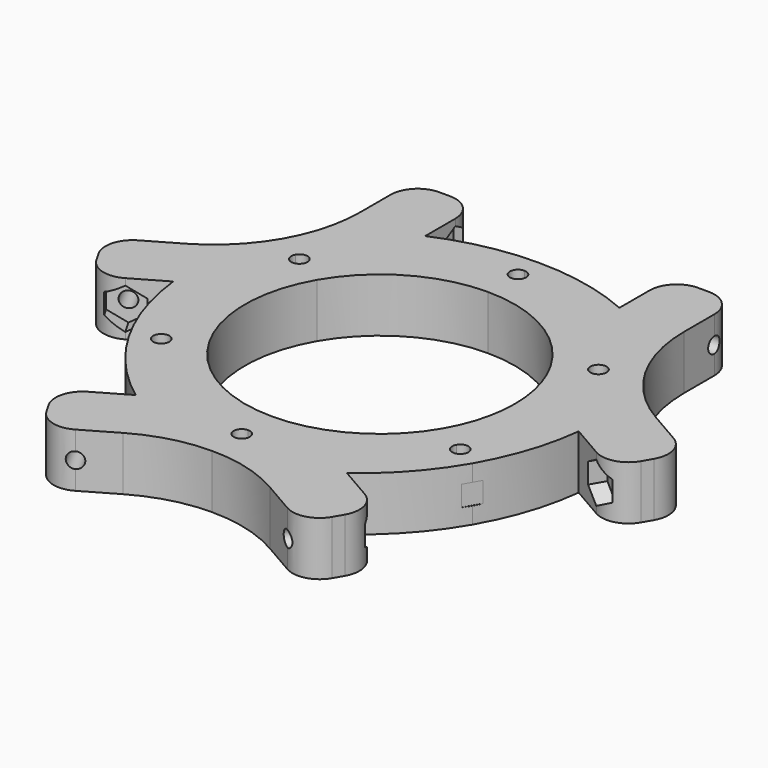
from build123d import *

# Parameters (mm, degrees)
F1_DEPTH      = 10
F2_R          = 1.45
F3_DEPTH      = 30
F3_DEPTH_BACK = 30
F4_ANGLE      = 120
F5_ANGLE      = 120
F7_T1_DEPTH   = 35
F8_DEPTH      = 21
F8_DEPTH_BACK = 21
F9_ANGLE      = 120
F10_ANGLE     = 120


# Not quite as in the source:
# - a fillet or chamfer that OpenCascade refuses, or shapes differently, is made with other operations: its cross-section is extruded or revolved along the edge and cut away or added
# - a feature names something its author has since deleted; it is built from what else it names


with BuildPart() as f1:
    # F0 (on Top) → F1 (new body)
    with BuildSketch(Plane.XY):
        with BuildLine():
            ThreePointArc((-21.6506350946, 12.5), (-12.5, 21.6506350946), (0, 25))
            Line((0, 25), (0, 30.5))
            ThreePointArc((0, 30.5), (-1.5, 32), (0, 33.5))
            Line((0, 33.5), (0, 36.7568187454))
            ThreePointArc((0, 36.7568187454), (-9.193933966, 35.8076028273), (-18, 33))
            Line((-18, 33), (-18, 45))
            Line((-18, 45), (-30, 45))
            Line((-30, 45), (-30, 33))
            ThreePointArc((-30, 33), (-30.9253753917, 25.9710760623), (-33.6384387633, 19.4211616751))
            Line((-33.6384387633, 19.4211616751), (-29.0118510268, 16.75))
            ThreePointArc((-29.0118510268, 16.75), (-27.3245843534, 17.4488887394), (-26.2128129211, 16))
            ThreePointArc((-26.2128129211, 16), (-26.2639241817, 15.6117714323), (-26.4137748154, 15.25))
            Line((-26.4137748154, 15.25), (-21.6506350946, 12.5))
        make_face()
        with BuildLine():
            ThreePointArc((0, -25), (-12.5, -21.6506350946), (-21.6506350946, -12.5))
            Line((-21.6506350946, -12.5), (-26.4137748154, -15.25))
            ThreePointArc((-26.4137748154, -15.25), (-26.2639241817, -15.6117714323), (-26.2128129211, -16))
            ThreePointArc((-26.2128129211, -16), (-27.3245843534, -17.4488887394), (-29.0118510268, -16.75))
            Line((-29.0118510268, -16.75), (-31.8323387958, -18.3784093727))
            ThreePointArc((-31.8323387958, -18.3784093727), (-26.413326714, -25.8659817889), (-19.5788383249, -32.0884572681))
            Line((-19.5788383249, -32.0884572681), (-29.9711431703, -38.0884572681))
            Line((-29.9711431703, -38.0884572681), (-23.9711431703, -48.4807621135))
            Line((-23.9711431703, -48.4807621135), (-13.5788383249, -42.4807621135))
            ThreePointArc((-13.5788383249, -42.4807621135), (-7.0289239377, -39.767698742), (0, -38.8423233502))
            Line((0, -38.8423233502), (0, -33.5))
            ThreePointArc((0, -33.5), (-1.5, -32), (0, -30.5))
            Line((0, -30.5), (0, -25))
        make_face()
        with BuildLine():
            Line((0, 30.5), (0, 25))
            ThreePointArc((0, 25), (12.5, 21.6506350946), (21.6506350946, 12.5))
            Line((21.6506350946, 12.5), (26.4137748154, 15.25))
            ThreePointArc((26.4137748154, 15.25), (26.9628129211, 17.2990381057), (29.0118510268, 16.75))
            Line((29.0118510268, 16.75), (33.6384387633, 19.4211616751))
            ThreePointArc((33.6384387633, 19.4211616751), (30.9253753917, 25.9710760623), (30, 33))
            Line((30, 33), (30, 45))
            Line((30, 45), (18, 45))
            Line((18, 45), (18, 33))
            ThreePointArc((18, 33), (9.193933966, 35.8076028273), (0, 36.7568187454))
            Line((0, 36.7568187454), (0, 33.5))
            ThreePointArc((0, 33.5), (1.0606601718, 33.0606601718), (1.5, 32))
            ThreePointArc((1.5, 32), (1.0606601718, 30.9393398282), (0, 30.5))
        make_face()
        with BuildLine():
            ThreePointArc((25, 0), (24.1481456572, -6.4704761276), (21.6506350946, -12.5))
            Line((21.6506350946, -12.5), (26.4137748154, -15.25))
            ThreePointArc((26.4137748154, -15.25), (28.1010414888, -14.5511112606), (29.2128129211, -16))
            ThreePointArc((29.2128129211, -16), (29.1617016605, -16.3882285677), (29.0118510268, -16.75))
            Line((29.0118510268, -16.75), (31.8323387958, -18.3784093727))
            ThreePointArc((31.8323387958, -18.3784093727), (35.6072606801, -9.9416210384), (37.5788383249, -0.9115427319))
            Line((37.5788383249, -0.9115427319), (47.9711431703, -6.9115427319))
            Line((47.9711431703, -6.9115427319), (53.9711431703, 3.4807621135))
            Line((53.9711431703, 3.4807621135), (43.5788383249, 9.4807621135))
            ThreePointArc((43.5788383249, 9.4807621135), (37.9542993294, 13.7966226797), (33.6384387633, 19.4211616751))
            Line((33.6384387633, 19.4211616751), (29.0118510268, 16.75))
            ThreePointArc((29.0118510268, 16.75), (29.1617016605, 16.3882285677), (29.2128129211, 16))
            ThreePointArc((29.2128129211, 16), (28.1010414888, 14.5511112606), (26.4137748154, 15.25))
            Line((26.4137748154, 15.25), (21.6506350946, 12.5))
            ThreePointArc((21.6506350946, 12.5), (24.1481456572, 6.4704761276), (25, 0))
        make_face()
        with BuildLine():
            Line((-26.4137748154, -15.25), (-21.6506350946, -12.5))
            ThreePointArc((-21.6506350946, -12.5), (-25, 0), (-21.6506350946, 12.5))
            Line((-21.6506350946, 12.5), (-26.4137748154, 15.25))
            ThreePointArc((-26.4137748154, 15.25), (-28.4628129211, 14.7009618943), (-29.0118510268, 16.75))
            Line((-29.0118510268, 16.75), (-33.6384387633, 19.4211616751))
            ThreePointArc((-33.6384387633, 19.4211616751), (-37.9542993294, 13.7966226797), (-43.5788383249, 9.4807621135))
            Line((-43.5788383249, 9.4807621135), (-53.9711431703, 3.4807621135))
            Line((-53.9711431703, 3.4807621135), (-47.9711431703, -6.9115427319))
            Line((-47.9711431703, -6.9115427319), (-37.5788383249, -0.9115427319))
            ThreePointArc((-37.5788383249, -0.9115427319), (-35.6072606801, -9.9416210384), (-31.8323387958, -18.3784093727))
            Line((-31.8323387958, -18.3784093727), (-29.0118510268, -16.75))
            ThreePointArc((-29.0118510268, -16.75), (-28.4628129211, -14.7009618943), (-26.4137748154, -15.25))
        make_face()
        with BuildLine():
            Line((26.4137748154, -15.25), (21.6506350946, -12.5))
            ThreePointArc((21.6506350946, -12.5), (12.5, -21.6506350946), (0, -25))
            Line((0, -25), (0, -30.5))
            ThreePointArc((0, -30.5), (1.0606601718, -30.9393398282), (1.5, -32))
            ThreePointArc((1.5, -32), (1.0606601718, -33.0606601718), (0, -33.5))
            Line((0, -33.5), (0, -38.8423233502))
            ThreePointArc((0, -38.8423233502), (7.0289239377, -39.767698742), (13.5788383249, -42.4807621135))
            Line((13.5788383249, -42.4807621135), (23.9711431703, -48.4807621135))
            Line((23.9711431703, -48.4807621135), (29.9711431703, -38.0884572681))
            Line((29.9711431703, -38.0884572681), (19.5788383249, -32.0884572681))
            ThreePointArc((19.5788383249, -32.0884572681), (26.413326714, -25.8659817889), (31.8323387958, -18.3784093727))
            Line((31.8323387958, -18.3784093727), (29.0118510268, -16.75))
            ThreePointArc((29.0118510268, -16.75), (26.9628129211, -17.2990381057), (26.4137748154, -15.25))
        make_face()
    extrude(amount=F1_DEPTH)


with BuildPart() as f3:
    # F2 (on Right) → F3 (new body, two sides)
    with BuildSketch(Plane.YZ) as f3_sk:
        with Locations((40, 5)):
            Circle(F2_R)
    extrude(amount=F3_DEPTH)
    extrude(f3_sk.sketch, amount=-F3_DEPTH_BACK)


with BuildPart() as f4_1:
    # F4: copy of F3
    add(f3.part.rotate(Axis((0, 0, 10), (0, 0, -1)), F4_ANGLE))


with BuildPart() as f5_1:
    # F5: copy of F4_1
    add(f4_1.part.rotate(Axis((0, 0, 10), (0, 0, -1)), F5_ANGLE))


with BuildPart() as f1_1:
    add(f1.part)

    # F6: cut F5_1, F3, F4_1
    add(f5_1.part, mode=Mode.SUBTRACT)
    add(f3.part, mode=Mode.SUBTRACT)
    add(f4_1.part, mode=Mode.SUBTRACT)

    # F7: fillet of radius 5 on 12 edges, made by hand

    # F7_s2 → F7_t1 (cut)
    with BuildSketch(Plane.XY.offset(-12.5)):
        with BuildLine():
            ThreePointArc((-26.4711431703, -44.1506350946), (-23.4351113769, -46.4802642261), (-19.6410161514, -45.9807621135))
            Line((-19.6410161514, -45.9807621135), (-23.9711431703, -48.4807621135))
            Line((-23.9711431703, -48.4807621135), (-26.4711431703, -44.1506350946))
        make_face()
        with BuildLine():
            ThreePointArc((19.6410161514, -45.9807621135), (23.4351113769, -46.4802642261), (26.4711431703, -44.1506350946))
            Line((26.4711431703, -44.1506350946), (23.9711431703, -48.4807621135))
            Line((23.9711431703, -48.4807621135), (19.6410161514, -45.9807621135))
        make_face()
        with BuildLine():
            ThreePointArc((51.4711431703, -0.8493649054), (51.9706452828, 2.9447303201), (49.6410161514, 5.9807621135))
            Line((49.6410161514, 5.9807621135), (53.9711431703, 3.4807621135))
            Line((53.9711431703, 3.4807621135), (51.4711431703, -0.8493649054))
        make_face()
        with BuildLine():
            ThreePointArc((30, 40), (28.5355339059, 43.5355339059), (25, 45))
            Line((25, 45), (30, 45))
            Line((30, 45), (30, 40))
        make_face()
        with BuildLine():
            ThreePointArc((-25, 45), (-28.5355339059, 43.5355339059), (-30, 40))
            Line((-30, 40), (-30, 45))
            Line((-30, 45), (-25, 45))
        make_face()
        with BuildLine():
            ThreePointArc((-49.6410161514, 5.9807621135), (-51.9706452828, 2.9447303201), (-51.4711431703, -0.8493649054))
            Line((-51.4711431703, -0.8493649054), (-53.9711431703, 3.4807621135))
            Line((-53.9711431703, 3.4807621135), (-49.6410161514, 5.9807621135))
        make_face()
        with BuildLine():
            ThreePointArc((27.4711431703, -42.418584287), (27.9706452828, -38.6244890615), (25.6410161514, -35.5884572681))
            Line((25.6410161514, -35.5884572681), (29.9711431703, -38.0884572681))
            Line((29.9711431703, -38.0884572681), (27.4711431703, -42.418584287))
        make_face()
        with BuildLine():
            ThreePointArc((43.6410161514, -4.4115427319), (47.4351113769, -4.9110448444), (50.4711431703, -2.581415713))
            Line((50.4711431703, -2.581415713), (47.9711431703, -6.9115427319))
            Line((47.9711431703, -6.9115427319), (43.6410161514, -4.4115427319))
        make_face()
        with BuildLine():
            ThreePointArc((23, 45), (19.4644660941, 43.5355339059), (18, 40))
            Line((18, 40), (18, 45))
            Line((18, 45), (23, 45))
        make_face()
        with BuildLine():
            ThreePointArc((-18, 40), (-19.4644660941, 43.5355339059), (-23, 45))
            Line((-23, 45), (-18, 45))
            Line((-18, 45), (-18, 40))
        make_face()
        with BuildLine():
            ThreePointArc((-50.4711431703, -2.581415713), (-47.4351113769, -4.9110448444), (-43.6410161514, -4.4115427319))
            Line((-43.6410161514, -4.4115427319), (-47.9711431703, -6.9115427319))
            Line((-47.9711431703, -6.9115427319), (-50.4711431703, -2.581415713))
        make_face()
        with BuildLine():
            ThreePointArc((-25.6410161514, -35.5884572681), (-27.9706452828, -38.6244890615), (-27.4711431703, -42.418584287))
            Line((-27.4711431703, -42.418584287), (-29.9711431703, -38.0884572681))
            Line((-29.9711431703, -38.0884572681), (-25.6410161514, -35.5884572681))
        make_face()
    extrude(amount=F7_T1_DEPTH, mode=Mode.SUBTRACT)


with BuildPart() as f8:
    # F2 (on Right) → F8 (new body, two sides)
    with BuildSketch(Plane.YZ) as f8_sk:
        Polygon((43.275, 3.1091778684), (43.275, 6.8908221316), (40, 8.7816442632), (36.725, 6.8908221316), (36.725, 3.1091778684), (40, 1.2183557368), align=None)
        with Locations((40, 5)):
            Circle(F2_R, mode=Mode.SUBTRACT)
    extrude(amount=F8_DEPTH)
    extrude(f8_sk.sketch, amount=-F8_DEPTH_BACK)


with BuildPart() as f9_1:
    # F9: copy of F8
    add(f8.part.rotate(Axis((0, 0, 10), (0, 0, -1)), F9_ANGLE))


with BuildPart() as f10_1:
    # F10: copy of F9_1
    add(f9_1.part.rotate(Axis((0, 0, 10), (0, 0, -1)), F10_ANGLE))


with BuildPart() as f1_2:
    add(f1_1.part)

    # F11: cut F8, F10_1, F9_1
    add(f8.part, mode=Mode.SUBTRACT)
    add(f10_1.part, mode=Mode.SUBTRACT)
    add(f9_1.part, mode=Mode.SUBTRACT)


solid = f1_2.part
